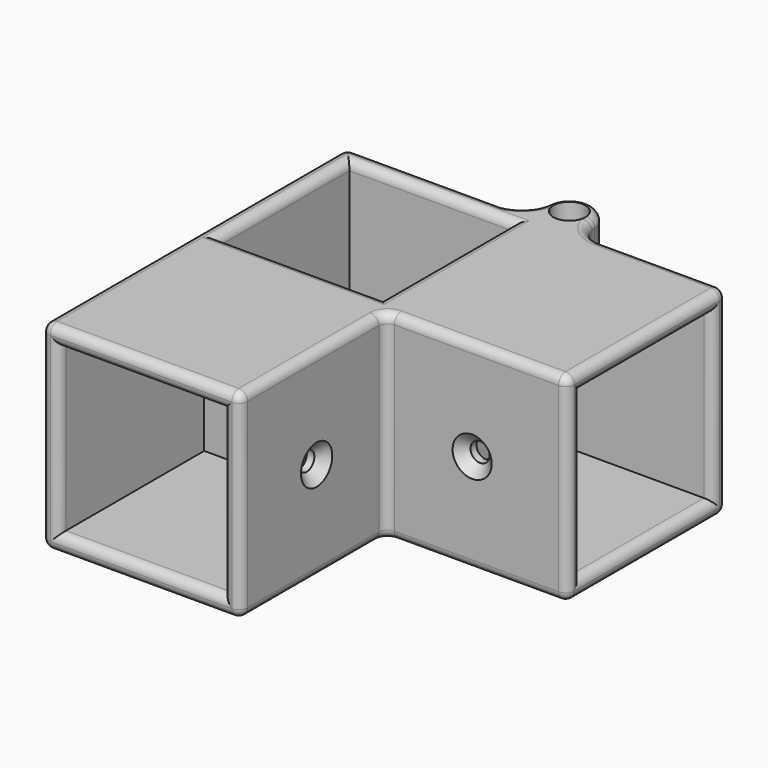
from build123d import *

# Parameters (mm, degrees)
F0_W                   = 34.2
F0_H                   = 34.2
F0_W_2                 = 28.2
F0_H_2                 = 28.2
F1_DEPTH               = 3
F2_DEPTH               = 31.2
F3_W                   = 34.2
F3_H                   = 34.2
F3_W_2                 = 28.2
F3_H_2                 = 28.2
F4_DEPTH               = 31.2
F5_W                   = 34.2
F5_H                   = 34.2
F5_W_2                 = 28.2
F5_H_2                 = 28.2
F6_DEPTH               = 31.2
F7_D                   = 3.3
F7_DEPTH               = 13.5
F7_CSINK_D             = 6.72
F7_CSINK_ANGLE         = 90
F7_TIP                 = 0.9914200214
F7_ON_F3_D             = 3.3
F7_ON_F3_DEPTH         = 13.5
F7_ON_F3_CSINK_D       = 6.72
F7_ON_F3_CSINK_ANGLE   = 90
F7_ON_F3_TIP           = 0.9914200214
F10_D                  = 3.3
F10_DEPTH              = 13.5
F10_CSINK_D            = 6.72
F10_CSINK_ANGLE        = 90
F10_TIP                = 0.9914200214
F10_ON_F8_D            = 3.3
F10_ON_F8_DEPTH        = 13.5
F10_ON_F8_CSINK_D      = 6.72
F10_ON_F8_CSINK_ANGLE  = 90
F10_ON_F8_TIP          = 0.9914200214
F13_D                  = 3.3
F13_DEPTH              = 13.5
F13_CSINK_D            = 6.72
F13_CSINK_ANGLE        = 90
F13_TIP                = 0.9914200214
F13_ON_F11_D           = 3.3
F13_ON_F11_DEPTH       = 13.5
F13_ON_F11_CSINK_D     = 6.72
F13_ON_F11_CSINK_ANGLE = 90
F13_ON_F11_TIP         = 0.9914200214
F15_DEPTH              = 34.2
F16_D                  = 5.5
F16_DEPTH              = 25
F16_TIP                = 1.6523667023
F17_R                  = 5
F18_R                  = 1.49999
F19_D                  = 3.3
F19_DEPTH              = 13.5
F19_CSINK_D            = 6.72
F19_CSINK_ANGLE        = 90
F19_TIP                = 0.9914200214


# Not quite as in the source:
# - a fillet or chamfer is up to 0.001 mm smaller than in the source, because OpenCascade refuses the exact size


with BuildPart() as f1:
    # F0 (on Top) → F1 (new body)
    with BuildSketch(Plane.XY):
        with Locations((-14.1, 14.1)):
            Rectangle(F0_W, F0_H)
        with Locations((-14.1, 14.1)):
            Rectangle(F0_W_2, F0_H_2, mode=Mode.SUBTRACT)
        with Locations((-14.1, 14.1)):
            Rectangle(F0_W_2, F0_H_2)
    extrude(amount=-F1_DEPTH)

    # F0 (on Top) → F2 (join)
    with BuildSketch(Plane.XY):
        with Locations((-14.1, 14.1)):
            Rectangle(F0_W, F0_H)
        with Locations((-14.1, 14.1)):
            Rectangle(F0_W_2, F0_H_2, mode=Mode.SUBTRACT)
    extrude(amount=F2_DEPTH)

    # F3 (on face) → F4 (join)
    with BuildSketch(Plane.XZ.offset(3)):
        with Locations((-14.1, 14.1)):
            Rectangle(F3_W, F3_H)
        with Locations((-14.1, 14.1)):
            Rectangle(F3_W_2, F3_H_2, mode=Mode.SUBTRACT)
    extrude(amount=F4_DEPTH)

    # F5 (on face) → F6 (join)
    with BuildSketch(Plane.YZ.offset(3)):
        with Locations((14.1, 14.1)):
            Rectangle(F5_W, F5_H)
        with Locations((14.1, 14.1)):
            Rectangle(F5_W_2, F5_H_2, mode=Mode.SUBTRACT)
    extrude(amount=F6_DEPTH)

    # F7
    with Locations(Plane.YZ.offset(3)):
        with Locations((14.1, 14.1)):
            CounterSinkHole(F7_D / 2, F7_CSINK_D / 2, depth=F7_DEPTH, counter_sink_angle=F7_CSINK_ANGLE)
            with Locations((0, 0, -(F7_DEPTH + F7_TIP / 2))):  # 118° drill point
                Cone(0, F7_D / 2, F7_TIP, mode=Mode.SUBTRACT)

    # F7 on F3
    with Locations(Plane.XZ.offset(3)):
        with Locations((-14.1, 14.1)):
            CounterSinkHole(F7_ON_F3_D / 2, F7_ON_F3_CSINK_D / 2, depth=F7_ON_F3_DEPTH, counter_sink_angle=F7_ON_F3_CSINK_ANGLE)
            with Locations((0, 0, -(F7_ON_F3_DEPTH + F7_ON_F3_TIP / 2))):  # 118° drill point
                Cone(0, F7_ON_F3_D / 2, F7_ON_F3_TIP, mode=Mode.SUBTRACT)

    # F10
    with Locations(Plane.XZ.offset(3)):
        with Locations((17.85, 14.1)):
            CounterSinkHole(F10_D / 2, F10_CSINK_D / 2, depth=F10_DEPTH, counter_sink_angle=F10_CSINK_ANGLE)
            with Locations((0, 0, -(F10_DEPTH + F10_TIP / 2))):  # 118° drill point
                Cone(0, F10_D / 2, F10_TIP, mode=Mode.SUBTRACT)

    # F10 on F8
    with Locations(Plane.YZ.offset(3)):
        with Locations((-17.85, 14.1)):
            CounterSinkHole(F10_ON_F8_D / 2, F10_ON_F8_CSINK_D / 2, depth=F10_ON_F8_DEPTH, counter_sink_angle=F10_ON_F8_CSINK_ANGLE)
            with Locations((0, 0, -(F10_ON_F8_DEPTH + F10_ON_F8_TIP / 2))):  # 118° drill point
                Cone(0, F10_ON_F8_D / 2, F10_ON_F8_TIP, mode=Mode.SUBTRACT)

    # F13
    with Locations(Plane(origin=(-31.2, 0, 0), x_dir=(0, -1, 0), z_dir=(-1, 0, 0))):
        with Locations((-14.15, 14.1)):
            CounterSinkHole(F13_D / 2, F13_CSINK_D / 2, depth=F13_DEPTH, counter_sink_angle=F13_CSINK_ANGLE)
            with Locations((0, 0, -(F13_DEPTH + F13_TIP / 2))):  # 118° drill point
                Cone(0, F13_D / 2, F13_TIP, mode=Mode.SUBTRACT)

    # F13 on F11
    with Locations(Plane(origin=(0, 31.2, 0), x_dir=(-1, 0, 0), z_dir=(0, 1, 0))):
        with Locations((14.15, 14.1)):
            CounterSinkHole(F13_ON_F11_D / 2, F13_ON_F11_CSINK_D / 2, depth=F13_ON_F11_DEPTH, counter_sink_angle=F13_ON_F11_CSINK_ANGLE)
            with Locations((0, 0, -(F13_ON_F11_DEPTH + F13_ON_F11_TIP / 2))):  # 118° drill point
                Cone(0, F13_ON_F11_D / 2, F13_ON_F11_TIP, mode=Mode.SUBTRACT)

    # F14 (on face) → F15 (join, through all)
    with BuildSketch(Plane.XY.offset(31.2)):
        with BuildLine():
            Line((8.0105462586, 31.2), (8.0105462586, 35.1999722305))
            ThreePointArc((8.0105462586, 35.1999722305), (4.0158124775, 39.1999687638), (0.0105601252, 35.2105046591))
            Line((0.0105601252, 35.2105046591), (0, 31.2))
            Line((0, 31.2), (8.0105462586, 31.2))
        make_face()
    extrude(amount=-F15_DEPTH)

    # F16
    with Locations(Plane.XY.offset(31.2)):
        with Locations((4.0105462586, 35.1999722305)):
            Hole(F16_D / 2, depth=F16_DEPTH)
            with Locations((0, 0, -(F16_DEPTH + F16_TIP / 2))):  # 118° drill point
                Cone(0, F16_D / 2, F16_TIP, mode=Mode.SUBTRACT)

    # F17
    f17_edges = [f1.edges().sort_by_distance(p)[0] for p in [
        (0, 31.2, 14.1),
        (8.010546, 31.2, 14.1),
    ]]
    fillet(f17_edges, radius=F17_R)

    # F18 (radius 1.5 in the source; OpenCascade refuses exactly that, so slightly less here)
    f18_edges = [f1.edges().sort_by_distance(p)[0] for p in [
        (-18.066861, 31.2, 31.2),
        (-14.1, 28.2, 31.2),
        (-18.066861, 31.2, -3),
        (23.577408, 31.2, -3),
        (34.2, 14.1, 31.2),
        (34.2, 31.2, 14.1),
        (34.2, 28.2, 14.1),
        (34.2, 14.1, 28.2),
        (34.2, 0, 14.1),
        (34.2, -3, 14.1),
        (34.2, 14.1, -3),
        (34.2, 14.1, 0),
        (18.6, -3, -3),
        (3, -3, 14.1),
        (18.6, -3, 31.2),
        (3, -18.6, 31.2),
        (3, -34.2, 14.1),
        (-14.1, -34.2, 0),
        (0, -34.2, 14.1),
        (-14.1, -34.2, 28.2),
        (-28.2, -34.2, 14.1),
        (-14.1, -34.2, -3),
        (-14.1, -34.2, 31.2),
        (-31.2, -34.2, 14.1),
        (-31.2, -1.5, 31.2),
        (-31.2, 31.2, 14.1),
        (-31.2, -1.5, -3),
        (0, 14.1, 31.2),
        (-14.1, 0, 31.2),
        (-28.2, 14.1, 31.2),
        (9.621488, 32.473215, -3),
        (4.010546, 39.199972, -3),
        (-1.600395, 32.473215, -3),
        (3, -18.6, -3),
        (23.577408, 31.2, 31.2),
        (9.621488, 32.473215, 31.2),
        (-1.600395, 32.473215, 31.2),
    ]]
    fillet(f18_edges, radius=F18_R)

    # F19
    with Locations(Plane.XY):
        with Locations((-14.1, 14.1)):
            CounterSinkHole(F19_D / 2, F19_CSINK_D / 2, depth=F19_DEPTH, counter_sink_angle=F19_CSINK_ANGLE)
            with Locations((0, 0, -(F19_DEPTH + F19_TIP / 2))):  # 118° drill point
                Cone(0, F19_D / 2, F19_TIP, mode=Mode.SUBTRACT)


solid = f1.part
